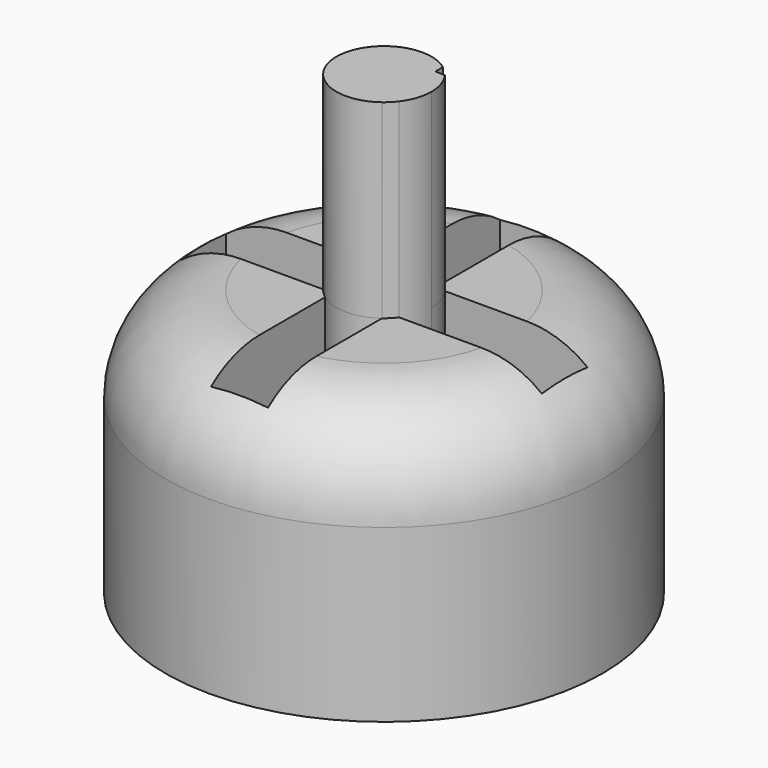
from build123d import *

# Parameters (mm, degrees)
F0_R     = 11.5
F1_DEPTH = 11
F2_R     = 11.5
F3_DEPTH = 3
F6_DEPTH = 10


# Not quite as in the source:
# - a fillet or chamfer that OpenCascade refuses, or shapes differently, is made with other operations: its cross-section is extruded or revolved along the edge and cut away or added


with BuildPart() as f1:
    # F0 (on Top) → F1 (new body)
    with BuildSketch(Plane.XY):
        Circle(F0_R)
        Polygon((9.5, 1.5), (9.5, -1.5), (1.5, -1.5), (1.5, -9.5), (-1.5, -9.5), (-1.5, -1.5), (-9.5, -1.5), (-9.5, 1.5), (-1.5, 1.5), (-1.5, 9.5), (1.5, 9.5), (1.5, 1.5), align=None, mode=Mode.SUBTRACT)
    extrude(amount=F1_DEPTH)

    # F2 (on face) → F3 (join)
    with BuildSketch(Plane.XY.offset(11)):
        Circle(F2_R)
        Polygon((1.5, 1.5), (9.5, 1.5), (9.5, -1.5), (1.5, -1.5), (1.5, -9.5), (-1.5, -9.5), (-1.5, -1.5), (-9.5, -1.5), (-9.5, 1.5), (-1.5, 1.5), (-1.5, 9.5), (1.5, 9.5), align=None, mode=Mode.SUBTRACT)
    extrude(amount=F3_DEPTH)

    # F4: fillet of radius 5 on 1 edges, made by hand

    # F4_s1 → F4_t2 (revolve, cut)
    with BuildSketch(Plane.XZ):
        with BuildLine():
            ThreePointArc((11.5, 9), (10.0355339059, 12.5355339059), (6.5, 14))
            Line((6.5, 14), (11.5, 14))
            Line((11.5, 14), (11.5, 9))
        make_face()
    revolve(axis=Axis((0, 0, 14), (0, 0, 1)), mode=Mode.SUBTRACT)

    # F5 (on face) → F6 (join, symmetric)
    with BuildSketch(Plane.XY.offset(14)):
        with BuildLine():
            ThreePointArc((2, -1.5), (2.3717082451, -0.790569415), (2.5, 0))
            ThreePointArc((2.5, 0), (2.3717082451, 0.790569415), (2, 1.5))
            Line((2, 1.5), (1.5, 1.5))
            Line((1.5, 1.5), (1.5, 2))
            ThreePointArc((1.5, 2), (0, 2.5), (-1.5, 2))
            Line((-1.5, 2), (-1.5, 1.5))
            Line((-1.5, 1.5), (-2, 1.5))
            ThreePointArc((-2, 1.5), (-2.5, 0), (-2, -1.5))
            Line((-2, -1.5), (-1.5, -1.5))
            Line((-1.5, -1.5), (-1.5, -2))
            ThreePointArc((-1.5, -2), (0, -2.5), (1.5, -2))
            Line((1.5, -2), (1.5, -1.5))
            Line((1.5, -1.5), (2, -1.5))
        make_face()
        with BuildLine():
            ThreePointArc((1.5, -2), (1.767766953, -1.767766953), (2, -1.5))
            Line((2, -1.5), (1.5, -1.5))
            Line((1.5, -1.5), (1.5, -2))
        make_face()
        with BuildLine():
            Line((-1.5, 1.5), (-1.5, 2))
            ThreePointArc((-1.5, 2), (-1.767766953, 1.767766953), (-2, 1.5))
            Line((-2, 1.5), (-1.5, 1.5))
        make_face()
        with BuildLine():
            ThreePointArc((-2, -1.5), (-1.767766953, -1.767766953), (-1.5, -2))
            Line((-1.5, -2), (-1.5, -1.5))
            Line((-1.5, -1.5), (-2, -1.5))
        make_face()
    extrude(amount=F6_DEPTH, both=True)


solid = f1.part
